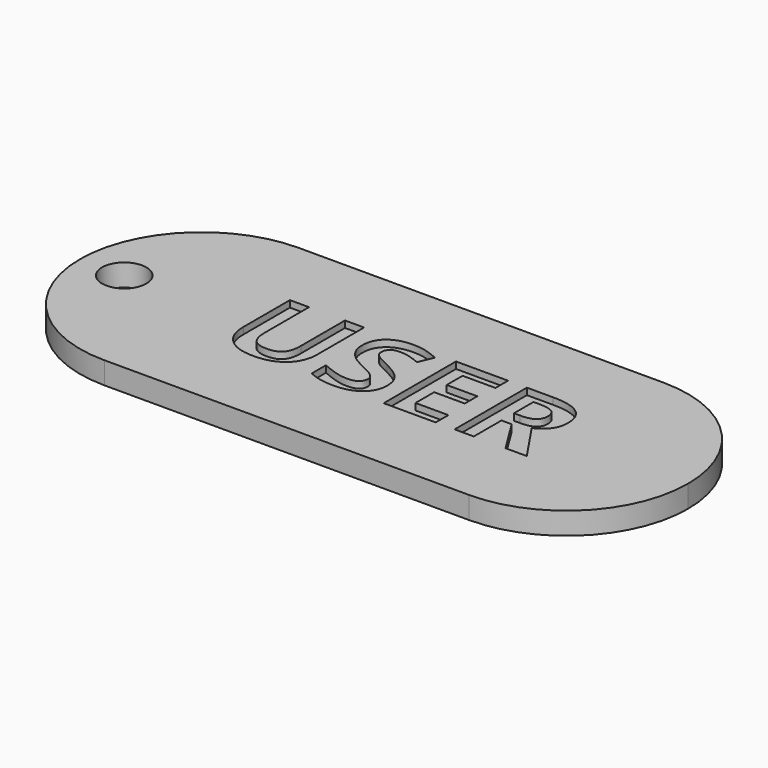
from build123d import *

# Parameters (mm, degrees)
F1_DEPTH     = 2
F2_D         = 4
F3_TEXT_SIZE = 11.4541666667
F4_DEPTH     = 0.6
F5_TEXT_SIZE = 8.3928922694
F6_DEPTH     = 0.6


# Not quite as in the source:
# - Text() gives the source's letters only with a copy of the font that has no kerning and outlines rounded to 1/6400 em; it was checked with that copy


with BuildPart() as f1:
    # F0 (on Top) → F1 (new body)
    with BuildSketch(Plane.XY):
        with BuildLine():
            Line((-16.5, 11), (-16.5, -11))
            ThreePointArc((-16.5, -11), (-8.7218254069, -7.7781745931), (-5.5, 0))
            ThreePointArc((-5.5, 0), (-8.7218254069, 7.7781745931), (-16.5, 11))
        make_face()
        with BuildLine():
            ThreePointArc((-16.5, 11), (-27.5, 0), (-16.5, -11))
            Line((-16.5, -11), (-16.5, 11))
        make_face()
        with BuildLine():
            ThreePointArc((16.5, 11), (5.5, 0), (16.5, -11))
            Line((16.5, -11), (16.5, 11))
        make_face()
        with BuildLine():
            Line((-16.5, -11), (16.5, -11))
            ThreePointArc((16.5, -11), (5.5, 0), (16.5, 11))
            Line((16.5, 11), (-16.5, 11))
            ThreePointArc((-16.5, 11), (-8.7218254069, 7.7781745931), (-5.5, 0))
            ThreePointArc((-5.5, 0), (-8.7218254069, -7.7781745931), (-16.5, -11))
        make_face()
        with BuildLine():
            Line((16.5, 11), (16.5, -11))
            ThreePointArc((16.5, -11), (24.2781745931, -7.7781745931), (27.5, 0))
            ThreePointArc((27.5, 0), (24.2781745931, 7.7781745931), (16.5, 11))
        make_face()
    extrude(amount=F1_DEPTH)

    # F2 (through all)
    with Locations(Plane(origin=(0, 0, 0), x_dir=(1, 0, 0), z_dir=(0, 0, -1))):
        with Locations((-23.5, 0)):
            Hole(F2_D / 2)

    # F3 (on face) → F4 (cut)
    with BuildSketch(Plane.XY.offset(2)):
        with Locations((-12.9812632978, -3.8063990197)):
            Text('USER', F3_TEXT_SIZE, font='Open Sans', font_style=FontStyle.BOLD, text_align=(TextAlign.LEFT, TextAlign.BOTTOM))
    extrude(amount=-F4_DEPTH, mode=Mode.SUBTRACT)

    # F5 (on face) → F6 (cut)
    with BuildSketch(Plane(origin=(0, 0, 0), x_dir=(1, 0, 0), z_dir=(0, 0, -1))):
        with Locations((-17.4145474226, -2.812036718)):
            Text('013241D9', F5_TEXT_SIZE, font='Open Sans', font_style=FontStyle.BOLD, text_align=(TextAlign.LEFT, TextAlign.BOTTOM))
    extrude(amount=-F6_DEPTH, mode=Mode.SUBTRACT)


solid = f1.part
